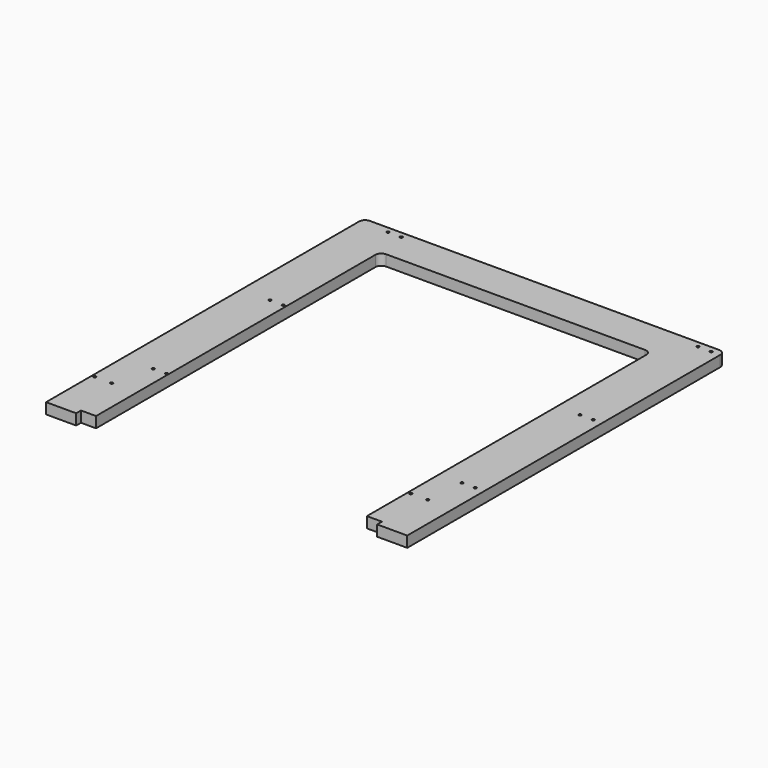
from build123d import *

# Parameters (mm, degrees)
F0_W     = 50
F0_H     = 10
F1_DEPTH = 18
F2_W     = 18
F2_H     = 50
F3_DEPTH = 10
F5_D     = 4.3
F6_R     = 10
F7_R     = 10


# Not quite as in the source:
# - a feature names something its author has since deleted; it is built from what else it names


with BuildPart() as f1:
    # F0 (on Top) → F1 (new body)
    with BuildSketch(Plane.XY):
        Polygon((600, 0), (0, 0), (0, -650), (50, -650), (75, -650), (75, -60), (525, -60), (525, -650), (550, -650), (600, -650), align=None)
        with Locations((25, -655)):
            Rectangle(F0_W, F0_H)
        with Locations((575, -655)):
            Rectangle(F0_W, F0_H)
    extrude(amount=F1_DEPTH)

    # F2 (on face) → F3 (cut)
    with BuildSketch(Plane(origin=(0, 0, 0), x_dir=(1, 0, 0), z_dir=(0, 0, -1))):
        with Locations((39, 590)):
            Rectangle(F2_W, F2_H)
        with Locations((39, 400)):
            Rectangle(F2_W, F2_H)
        with Locations((39, 200)):
            Rectangle(F2_W, F2_H)
        with Locations((561, 200)):
            Rectangle(F2_W, F2_H)
        with Locations((561, 400)):
            Rectangle(F2_W, F2_H)
        with Locations((561, 590)):
            Rectangle(F2_W, F2_H)
    extrude(amount=-F3_DEPTH, mode=Mode.SUBTRACT)

    # F5 (through all)
    with Locations(Plane.XY.offset(18)):
        with Locations((563, -10), (585, -10), (563, -255), (563, -500), (585, -500), (585, -255), (48, -10), (70, -10), (48, -255), (70, -255), (50, -500), (72, -500), (530, -565), (558, -565), (5, -565), (33, -565)):
            Hole(F5_D / 2)

    # F6
    f6_edges = [f1.edges().sort_by_distance(p)[0] for p in [
        (75, -60, 9),
        (525, -60, 9),
    ]]
    fillet(f6_edges, radius=F6_R)

    # F7
    f7_edges = [f1.edges().sort_by_distance(p)[0] for p in [
        (600, 0, 9),
        (0, 0, 9),
    ]]
    fillet(f7_edges, radius=F7_R)


solid = f1.part
